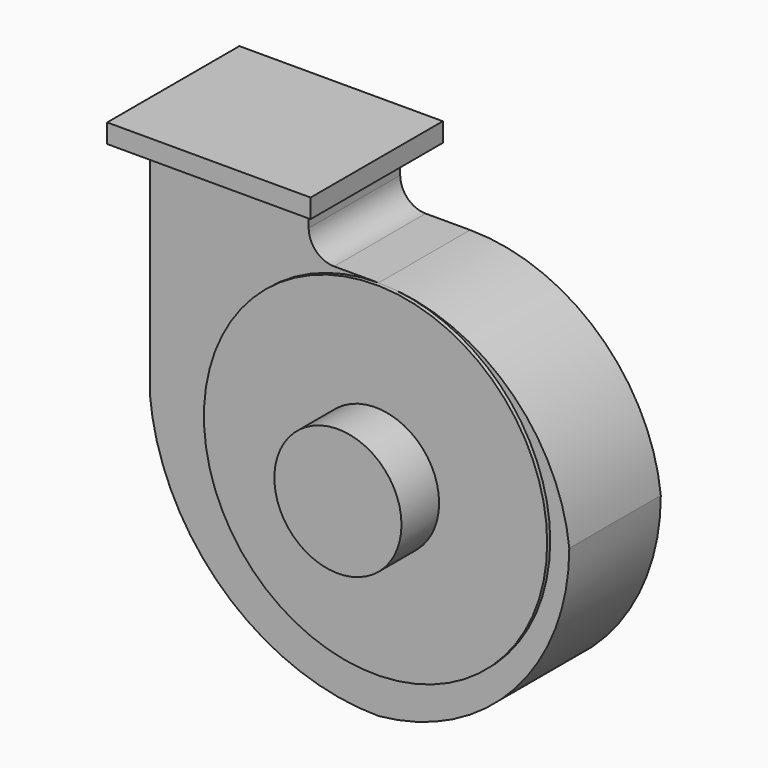
from build123d import *
from build123d import SkipClean  # not in build123d's __all__

# Parameters (mm, degrees)
F0_R     = 63.5
F2_DEPTH = 1270
F3_DEPTH = 1270
F4_DEPTH = 1270
F1_W     = 50.8
F1_H     = 127
F5_DEPTH = 1270
F6_DEPTH = 60.96


with BuildPart() as f2:
    # F0 (on Front) → F2 (new body, symmetric)
    with BuildSketch(Plane.XZ):
        Polygon((-228.6, 222.25), (-69.85, 222.25), (-47.625, 222.25), (-47.625, 241.3), (-250.825, 241.3), (-250.825, 222.25), align=None)
        with BuildLine():
            ThreePointArc((190.5, 0), (128.1457690484, 122.2758544982), (0, 171.45))
            Line((0, 171.45), (-44.45, 171.45))
            ThreePointArc((-44.45, 171.45), (-62.4105122421, 178.8894877579), (-69.85, 196.85))
            Line((-69.85, 196.85), (-69.85, 222.25))
            Line((-69.85, 222.25), (-228.6, 222.25))
            Line((-228.6, 222.25), (-228.6, 0))
            ThreePointArc((-228.6, 0), (-155.0557661778, -149.2358358304), (0, -209.55))
            ThreePointArc((0, -209.55), (135.7567353, -141.5993048182), (190.5, 0))
        make_face()
        with BuildLine():
            ThreePointArc((0, 171.45), (121.2334576344, 121.2334576344), (171.45, 0))
            ThreePointArc((171.45, 0), (-121.2334576344, -121.2334576344), (0, 171.45))
        make_face(mode=Mode.SUBTRACT)
        with BuildLine():
            ThreePointArc((0, 171.45), (-121.2334576344, -121.2334576344), (171.45, 0))
            ThreePointArc((171.45, 0), (121.2334576344, 121.2334576344), (0, 171.45))
        make_face()
        Circle(F0_R, mode=Mode.SUBTRACT)
        Circle(F0_R)
    extrude(amount=F2_DEPTH, both=True)

    # F1 (on Right) → F3 (intersect, symmetric)
    with BuildSketch(Plane.YZ):
        Polygon((-57.15, 222.25), (57.15, 222.25), (82.55, 222.25), (82.55, 241.3), (-82.55, 241.3), (-82.55, 222.25), align=None)
        Polygon((-57.15, -63.5), (-57.15, -209.55), (57.15, -209.55), (57.15, 222.25), (-57.15, 222.25), (-57.15, 63.5), align=None)
    extrude(amount=F3_DEPTH, both=True, mode=Mode.INTERSECT)



with BuildPart() as f4:
    # F0 (on Front) → F4 (new body, symmetric)
    with BuildSketch(Plane.XZ):
        Circle(F0_R)
    extrude(amount=F4_DEPTH, both=True)

    # F1 (on Right) → F5 (intersect, symmetric)
    with BuildSketch(Plane.YZ):
        with Locations((-82.55, 0)):
            Rectangle(F1_W, F1_H)
    extrude(amount=F5_DEPTH, both=True, mode=Mode.INTERSECT)


with BuildPart() as f2_1:
    add(f2.part, clean=False)

    with SkipClean():  # cleaning this boolean's faces spoils the solid; the shape is the same uncleaned
        add(f4.part)  # F6 merges F4
    # F0 (on Front) → F6 (join)
    with BuildSketch(Plane.XZ):
        with BuildLine():
            ThreePointArc((0, 171.45), (-121.2334576344, -121.2334576344), (171.45, 0))
            ThreePointArc((171.45, 0), (121.2334576344, 121.2334576344), (0, 171.45))
        make_face()
        Circle(F0_R, mode=Mode.SUBTRACT)
    with SkipClean():  # cleaning this boolean's faces spoils the solid; the shape is the same uncleaned
        extrude(amount=F6_DEPTH)


solid = f2_1.part
